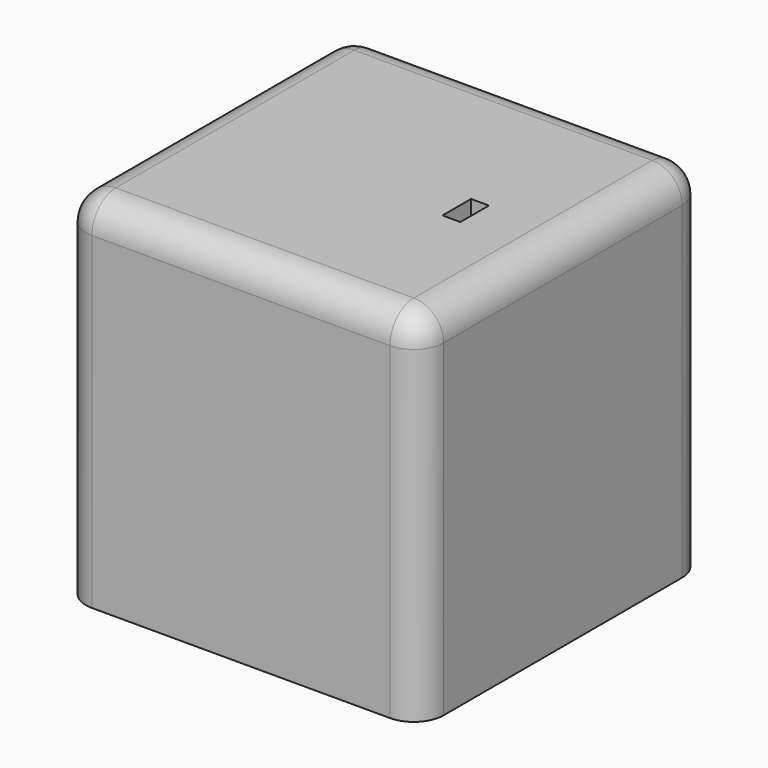
from build123d import *

# Parameters (mm, degrees)
F0_W     = 60
F0_H     = 60
F1_DEPTH = 60
F2_R     = 5
F3_T     = 5
F4_W     = 3
F4_H     = 6
F5_DEPTH = 25


# Not quite as in the source:
# - a shell that OpenCascade refuses in one call is made with other operations: the cavity is built on its own and cut out


with BuildPart() as f1:
    # F0 (on Top) → F1 (new body)
    with BuildSketch(Plane.XY):
        with Locations((-4.3964601223, -1.0684304871)):
            Rectangle(F0_W, F0_H)
    extrude(amount=F1_DEPTH)

    # F2
    f2_edges = [f1.edges().sort_by_distance(p)[0] for p in [
        (25.60354, 28.93157, 30),
        (-4.39646, 28.93157, 60),
        (-34.39646, 28.93157, 30),
        (-34.39646, -1.06843, 60),
        (-34.39646, -31.06843, 30),
        (-4.39646, -31.06843, 60),
        (25.60354, -31.06843, 30),
        (25.60354, -1.06843, 60),
    ]]
    fillet(f2_edges, radius=F2_R)

    # F3: shell of thickness 5, made by hand


with BuildPart() as f3_core1:
    # F3_t2: copy of F1
    add(f1.part)

    # the walls: a layer under each face that stays
    f3_faces = [f3_core1.faces().sort_by_distance(p)[0] for p in [
        (-4.3964601223, 28.9315695129, 27.5),
        (25.6035398777, -1.0684304871, 27.5),
        (-34.3964601223, -1.0684304871, 27.5),
        (-4.3964601223, -31.0684304871, 27.5),
        (-4.3964601223, -1.0684304871, 60),
    ]]
    thicken(f3_faces, amount=-F3_T, mode=Mode.SUBTRACT)


with BuildPart() as f1_1:
    add(f1.part)

    # what is left inside the walls is the cavity
    f3_cavity = [f3_core1.part.solids().sort_by_distance(p)[0] for p in [
        (20.55354, -1.06843, 36.666667),
    ]]
    add(f3_cavity, mode=Mode.SUBTRACT)

    # F4 (on face) → F5 (cut)
    with BuildSketch(Plane.XY.offset(60)):
        with Locations((10.4050671086, -2.4284604266)):
            Rectangle(F4_W, F4_H)
    extrude(amount=-F5_DEPTH, mode=Mode.SUBTRACT)


solid = f1_1.part
